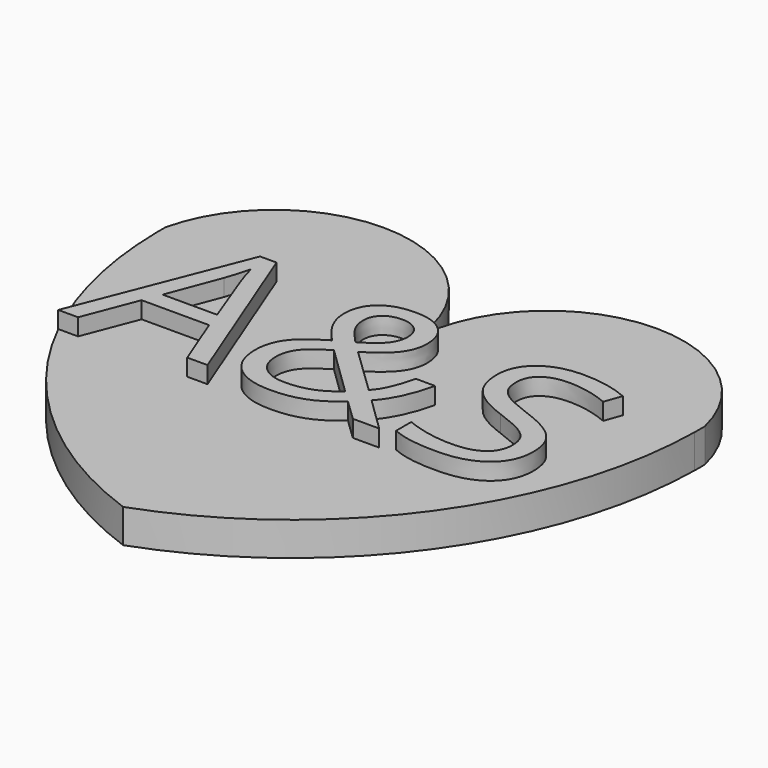
from build123d import *

# Parameters (mm, degrees)
F1_DEPTH     = 6.35
F2_TEXT_SIZE = 44.4494855384
F3_DEPTH     = 3.175


# Not quite as in the source:
# - Text() gives the source's letters only with a copy of the font that has no kerning and outlines rounded to 1/6400 em; it was checked with that copy


with BuildPart() as f1:
    # F0 (on Top) → F1 (new body)
    with BuildSketch(Plane.XY):
        with BuildLine():
            ThreePointArc((0, 16.9333333333), (-22.8108419546, 42.4985521958), (-50.8, 22.7369237691))
            Line((-50.8, 22.7369237691), (-50.8, 20.3336643665))
            ThreePointArc((-50.8, 20.3336643665), (-36.4904619218, -23.1534046082), (0, -50.8))
            Line((0, -50.8), (0, 16.9333333333))
        make_face()
        with BuildLine():
            Line((-50.8, 20.3336643665), (-50.8, 22.7369237691))
            ThreePointArc((-50.8, 22.7369237691), (-50.8093894254, 21.5352940678), (-50.8, 20.3336643665))
        make_face()
        with BuildLine():
            ThreePointArc((50.8, 20.3336643665), (50.8093894254, 21.5352940678), (50.8, 22.7369237691))
            Line((50.8, 22.7369237691), (50.8, 20.3336643665))
        make_face()
        with BuildLine():
            Line((50.8, 20.3336643665), (50.8, 22.7369237691))
            ThreePointArc((50.8, 22.7369237691), (22.8108419546, 42.4985521958), (0, 16.9333333333))
            Line((0, 16.9333333333), (0, -50.8))
            ThreePointArc((0, -50.8), (36.4904619218, -23.1534046082), (50.8, 20.3336643665))
        make_face()
    extrude(amount=F1_DEPTH)

    # F2 (on face) → F3 (join)
    with BuildSketch(Plane.XY.offset(6.35)):
        with Locations((-42.8625, -12.5088108348)):
            Text('A&S', F2_TEXT_SIZE, font='Open Sans', text_align=(TextAlign.LEFT, TextAlign.BOTTOM))
    extrude(amount=F3_DEPTH)


solid = f1.part
